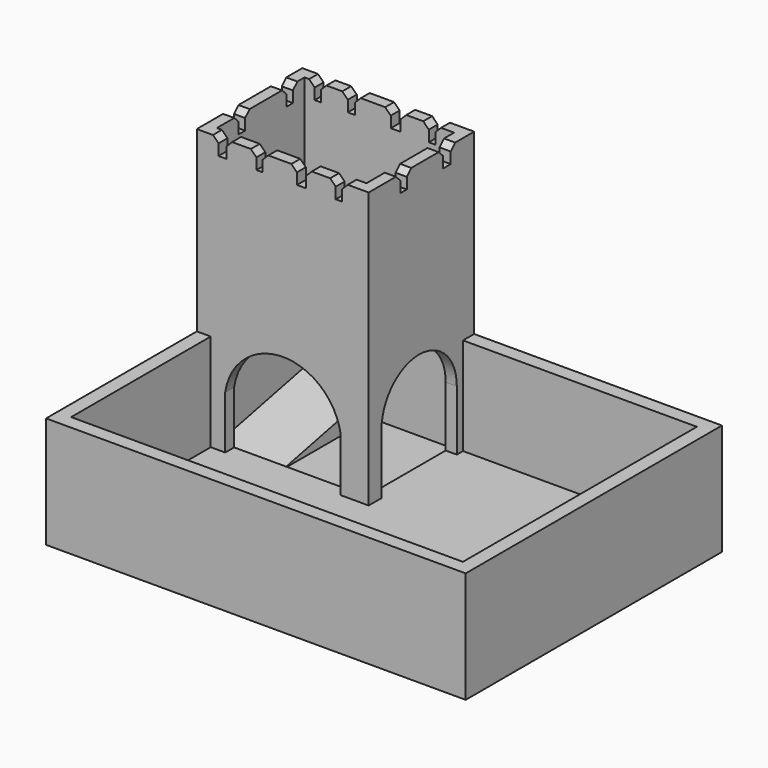
from build123d import *

# Parameters (mm, degrees)
F0_W         = 95.7279466093
F0_H         = 73.0648599565
F1_DEPTH     = 25.4
F2_T         = -3.175
F3_W         = 36.0267900012
F3_H         = 26.902483505
F4_DEPTH     = 22.225
F6_DEPTH     = 38.1
F7_T         = 2.54
F7_T3_DEPTH  = 8.255
F7_T5_DEPTH  = 8.255
F7_T7_DEPTH  = 27.305
F7_T9_DEPTH  = 31.982483505
F7_T11_DEPTH = 41.1067900012
F7_T13_DEPTH = 58.431156608
F7_T15_DEPTH = 71.7948599565
F7_T17_DEPTH = 94.4579466093
F7_T19_DEPTH = 44.8923764515
F8_W         = 26.3507906348
F8_H         = 12.0985915035
F9_DEPTH     = 3.175
F10_W        = 21.4841477573
F10_H        = 13.7384773314
F11_DEPTH    = 3.175
F13_W        = 1.8280372024
F13_H        = 2.54
F13_W_2      = 1.4438778162
F13_W_3      = 1.4618895948
F13_W_4      = 2.1120999008
F13_W_5      = 2.54
F13_H_2      = 1.8293876201
F13_H_3      = 1.8326565623
F13_W_6      = 1.4120712876
F13_W_7      = 1.6781240702
F13_W_8      = 2.2645629942
F13_W_9      = 1.5091551468
F13_H_4      = 2.1763034165
F13_H_5      = 1.8344689161
F14_DEPTH    = 1.27
F15_DEPTH    = 2.54
F16_SIZE     = 1.27
F17_SIZE     = 1.27
F18_SIZE     = 1.27
F19_SIZE     = 1.27
F20_DEPTH    = 15.24


# Not quite as in the source:
# - a shell that OpenCascade refuses in one call is made with other operations: the cavity is built on its own and cut out


with BuildPart() as f1:
    # F0 (on Top) → F1 (new body)
    with BuildSketch(Plane.XY):
        with Locations((3.9161536843, 6.8996157497)):
            Rectangle(F0_W, F0_H)
    extrude(amount=F1_DEPTH)

    # F2
    f2_openings = [f1.faces().sort_by_distance(p)[0] for p in [
        (3.916154, 6.899616, 25.4),
    ]]
    offset(amount=F2_T, openings=f2_openings)

    # F3 (on face) → F4 (join)
    with BuildSketch(Plane.XY.offset(3.175)):
        with Locations((-22.7594246197, 26.8058039755)):
            Rectangle(F3_W, F3_H)
    extrude(amount=F4_DEPTH)

    # F5 (on face) → F6 (join)
    with BuildSketch(Plane.XY.offset(25.4)):
        Polygon((-43.9478196204, 13.354562223), (-40.7728196204, 13.354562223), (-4.7460296191, 13.354562223), (-4.7460296191, 40.257045728), (-4.7460296191, 43.432045728), (-43.9478196204, 43.432045728), align=None)
    extrude(amount=F6_DEPTH)

    # F7: shell of thickness 2.54, made by hand


with BuildPart() as f7_core1:
    # F7_t2: copy of F1
    add(f1.part)

    # the walls: a layer under each face that stays
    f7_faces = [f7_core1.faces().sort_by_distance(p)[0] for p in [
        (-43.9478196204, 31.2545690686, 52.9166666667),
        (3.9161536843, 6.8996157497, 0),
        (51.7801269889, 6.8996157497, 12.7),
        (3.9161536843, -29.6328142285, 12.7),
        (-40.7568880667, -27.1973188967, 25.4),
        (-4.7460296191, 28.3933039755, 33.3375),
        (3.9161536843, 6.8996157497, 3.175),
        (21.9295486849, 40.257045728, 14.2875),
        (48.6051269889, 6.8996157497, 14.2875),
        (3.9161536843, -26.4578142285, 14.2875),
        (-40.7728196204, -6.5516260028, 14.2875),
        (-24.3469246197, 13.354562223, 33.3375),
        (35.8254692207, 43.432045728, 10.5833333333),
    ]]
    thicken(f7_faces, amount=-F7_T, mode=Mode.SUBTRACT)

    # F7_s4 → F7_t3 (cut)
    with BuildSketch(Plane.YZ.offset(-46.4878196204)):
        Polygon((13.329162223, 25.4254), (13.354562223, 22.86), (15.894562223, 22.86), (15.894562223, 25.4), align=None)
    extrude(amount=F7_T3_DEPTH, mode=Mode.SUBTRACT)

    # F7_s6 → F7_t5 (cut)
    with BuildSketch(Plane.XZ.offset(-45.972045728)):
        Polygon((-4.7206296191, 25.4254), (-4.7460296191, 22.86), (-7.2860296191, 22.86), (-7.2860296191, 25.4), align=None)
    extrude(amount=F7_T5_DEPTH, mode=Mode.SUBTRACT)

    # F7_s8 → F7_t7 (cut)
    with BuildSketch(Plane.XY.offset(0.635)):
        Polygon((-4.7206296191, 40.231645728), (-7.2860296191, 40.257045728), (-7.2860296191, 42.797045728), (-4.7460296191, 42.797045728), align=None)
        Polygon((48.5797269889, 40.231645728), (48.6051269889, 42.797045728), (51.1451269889, 42.797045728), (51.1451269889, 40.257045728), align=None)
        Polygon((48.5797269889, -26.4324142285), (51.1451269889, -26.4578142285), (51.1451269889, -28.9978142285), (48.6051269889, -28.9978142285), align=None)
        Polygon((-40.7474196204, -26.4324142285), (-40.7728196204, -28.9978142285), (-43.3128196204, -28.9978142285), (-43.3128196204, -26.4578142285), align=None)
        Polygon((-40.7474196204, 13.329162223), (-43.3128196204, 13.354562223), (-43.3128196204, 15.894562223), (-40.7728196204, 15.894562223), align=None)
    extrude(amount=F7_T7_DEPTH, mode=Mode.SUBTRACT)

    # F7_s10 → F7_t9 (cut)
    with BuildSketch(Plane.XZ.offset(-42.797045728)):
        Polygon((-4.7206296191, 3.2004), (-7.2860296191, 3.175), (-7.2860296191, 0.635), (-4.7460296191, 0.635), align=None)
    extrude(amount=F7_T9_DEPTH, mode=Mode.SUBTRACT)

    # F7_s12 → F7_t11 (cut)
    with BuildSketch(Plane.YZ.offset(-43.3128196204)):
        Polygon((13.329162223, 3.2004), (13.354562223, 0.635), (15.894562223, 0.635), (15.894562223, 3.175), align=None)
    extrude(amount=F7_T11_DEPTH, mode=Mode.SUBTRACT)

    # F7_s14 → F7_t13 (cut)
    with BuildSketch(Plane.YZ.offset(-7.2860296191)):
        Polygon((40.231645728, 3.2004), (40.257045728, 0.635), (42.797045728, 0.635), (42.797045728, 3.175), align=None)
    extrude(amount=F7_T13_DEPTH, mode=Mode.SUBTRACT)

    # F7_s16 → F7_t15 (cut)
    with BuildSketch(Plane.XZ.offset(-42.797045728)):
        Polygon((48.5797269889, 3.2004), (48.6051269889, 0.635), (51.1451269889, 0.635), (51.1451269889, 3.175), align=None)
    extrude(amount=F7_T15_DEPTH, mode=Mode.SUBTRACT)

    # F7_s18 → F7_t17 (cut)
    with BuildSketch(Plane.YZ.offset(-43.3128196204)):
        Polygon((-26.4324142285, 3.2004), (-26.4578142285, 0.635), (-28.9978142285, 0.635), (-28.9978142285, 3.175), align=None)
    extrude(amount=F7_T17_DEPTH, mode=Mode.SUBTRACT)

    # F7_s20 → F7_t19 (cut)
    with BuildSketch(Plane.XZ.offset(-15.894562223)):
        Polygon((-40.7474196204, 3.2004), (-40.7728196204, 0.635), (-43.3128196204, 0.635), (-43.3128196204, 3.175), align=None)
    extrude(amount=F7_T19_DEPTH, mode=Mode.SUBTRACT)


with BuildPart() as f1_1:
    add(f1.part)

    # what is left inside the walls is the cavity
    f7_cavity = [f7_core1.part.solids().sort_by_distance(p)[0] for p in [
        (-24.346925, 40.866646, 43.18),
    ]]
    add(f7_cavity, mode=Mode.SUBTRACT)

    # F8 (on face) → F9 (cut)
    with BuildSketch(Plane.XZ.offset(-13.354562223)):
        with BuildLine():
            ThreePointArc((-11.1161526293, 15.2735915035), (-24.2915479466, 26.6703128698), (-37.466943264, 15.2735915035))
            Line((-37.466943264, 15.2735915035), (-11.1161526293, 15.2735915035))
        make_face()
        with Locations((-24.2915479466, 9.2242957518)):
            Rectangle(F8_W, F8_H)
    extrude(amount=-F9_DEPTH, mode=Mode.SUBTRACT)

    # F10 (on face) → F11 (cut)
    with BuildSketch(Plane.YZ.offset(-4.7460296191)):
        with BuildLine():
            Line((17.0049779117, 16.9134773314), (38.489125669, 16.9134773314))
            ThreePointArc((38.489125669, 16.9134773314), (27.7470517904, 27.65555121), (17.0049779117, 16.9134773314))
        make_face()
        with Locations((27.7470517904, 10.0442386657)):
            Rectangle(F10_W, F10_H)
    extrude(amount=-F11_DEPTH, mode=Mode.SUBTRACT)

    # F13 (on face) → F14 (cut)
    with BuildSketch(Plane.XY.offset(63.5)):
        with Locations((-38.0768813193, 14.624562223)):
            Rectangle(F13_W, F13_H)
        with Locations((-29.6358391643, 14.624562223)):
            Rectangle(F13_W_2, F13_H)
        with Locations((-11.5280598402, 14.624562223)):
            Rectangle(F13_W_3, F13_H)
        with Locations((-20.0523110107, 14.624562223)):
            Rectangle(F13_W_4, F13_H)
        with Locations((-42.6778196204, 23.0370378122)):
            Rectangle(F13_W_5, F13_H_2)
        with Locations((-42.6778196204, 36.6639345884)):
            Rectangle(F13_W_5, F13_H_3)
        with Locations((-38.3811965585, 42.162045728)):
            Rectangle(F13_W_6, F13_H)
        with Locations((-30.6867770851, 42.162045728)):
            Rectangle(F13_W_7, F13_H)
        with Locations((-20.6000227481, 42.162045728)):
            Rectangle(F13_W_8, F13_H)
        with Locations((-12.2982370667, 42.162045728)):
            Rectangle(F13_W_9, F13_H)
        with Locations((-6.0160296191, 35.6560815126)):
            Rectangle(F13_W_5, F13_H_4)
        with Locations((-6.0160296191, 23.3017643914)):
            Rectangle(F13_W_5, F13_H_5)
    extrude(amount=-F14_DEPTH, mode=Mode.SUBTRACT)

    # F15 (add): faces of the model
    f15_faces = [f1_1.faces().sort_by_distance(p)[0] for p in [
        (-6.8630827973, 16.9610565444, 63.5),
        (-6.0160296191, 29.3934643269, 63.5),
        (-7.3381229169, 40.8948611138, 63.5),
        (-16.2602779455, 42.162045728, 63.5),
        (-25.7900096476, 42.162045728, 63.5),
        (-34.6005000174, 42.162045728, 63.5),
        (-41.9877249706, 40.9763533581, 63.5),
        (-42.6778196204, 29.8496689647, 63.5),
        (-42.1422453408, 17.0655675422, 63.5),
        (-33.7603203952, 14.624562223, 63.5),
        (-25.0111306086, 14.624562223, 63.5),
        (-15.6276328489, 14.624562223, 63.5),
    ]]
    extrude(f15_faces, amount=F15_DEPTH)

    # F16
    f16_edges = [f1_1.edges().sort_by_distance(p)[0] for p in [
        (-10.797115, 14.624562, 66.04),
        (-12.259005, 14.624562, 66.04),
    ]]
    chamfer(f16_edges, length=F16_SIZE)

    # F17
    f17_edges = [f1_1.edges().sort_by_distance(p)[0] for p in [
        (-6.01603, 22.38453, 66.04),
        (-6.01603, 24.218999, 66.04),
        (-6.01603, 34.56793, 66.04),
        (-6.01603, 36.744233, 66.04),
    ]]
    chamfer(f17_edges, length=F17_SIZE)

    # F18
    f18_edges = [f1_1.edges().sort_by_distance(p)[0] for p in [
        (-11.543659, 42.162046, 66.04),
        (-13.052815, 42.162046, 66.04),
        (-19.467741, 42.162046, 66.04),
        (-21.732304, 42.162046, 66.04),
        (-39.087232, 42.162046, 66.04),
        (-37.675161, 42.162046, 66.04),
        (-31.525839, 42.162046, 66.04),
        (-29.847715, 42.162046, 66.04),
    ]]
    chamfer(f18_edges, length=F18_SIZE)

    # F19
    f19_edges = [f1_1.edges().sort_by_distance(p)[0] for p in [
        (-42.67782, 37.580263, 66.04),
        (-42.67782, 35.747606, 66.04),
        (-42.67782, 23.951732, 66.04),
        (-42.67782, 22.122344, 66.04),
        (-38.9909, 14.624562, 66.04),
        (-37.162863, 14.624562, 66.04),
        (-30.357778, 14.624562, 66.04),
        (-28.9139, 14.624562, 66.04),
        (-21.108361, 14.624562, 66.04),
        (-18.996261, 14.624562, 66.04),
    ]]
    chamfer(f19_edges, length=F19_SIZE)

    # F12 (on face) → F20 (join)
    with BuildSketch(Plane.YZ.offset(-41.4078196204)):
        Polygon((40.892045728, 2.54), (40.892045728, 7.8878998756), (15.894562223, 2.54), align=None)
    extrude(amount=F20_DEPTH)


solid = f1_1.part
